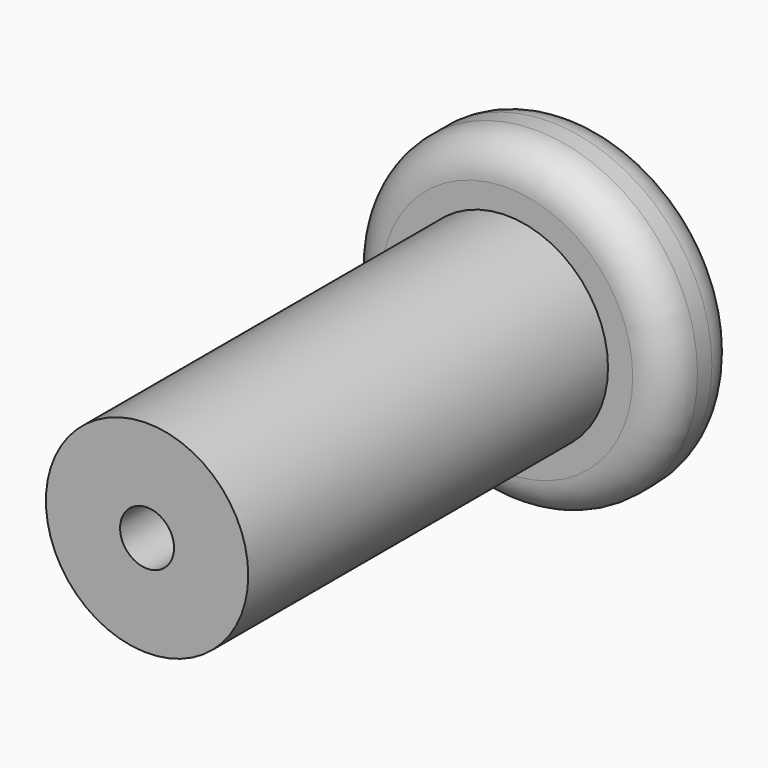
from build123d import *

# Parameters (mm, degrees)
F0_R     = 22.86
F0_R_2   = 14.2875
F2_DEPTH = 12.7
F3_R     = 5.08
F0_R_3   = 3.81
F5_DEPTH = 76.2


# Not quite as in the source:
# - the program builds the solid bodies; features that only make, move or delete a surface that nothing else refers to are left out


with BuildPart() as f2:
    # F0 (on Front) → F2 (new body)
    with BuildSketch(Plane.XZ):
        Circle(F0_R)
        Circle(F0_R_2, mode=Mode.SUBTRACT)
    extrude(amount=F2_DEPTH)

    # F3
    f3_edges = [f2.edges().sort_by_distance(p)[0] for p in [
        (-22.86, 0, 0),
        (-22.86, -12.7, 0),
    ]]
    fillet(f3_edges, radius=F3_R)

    # F0 (on Front) → F5 (join)
    with BuildSketch(Plane.XZ):
        Circle(F0_R_2)
        Circle(F0_R_3, mode=Mode.SUBTRACT)
    extrude(amount=F5_DEPTH)


solid = f2.part
